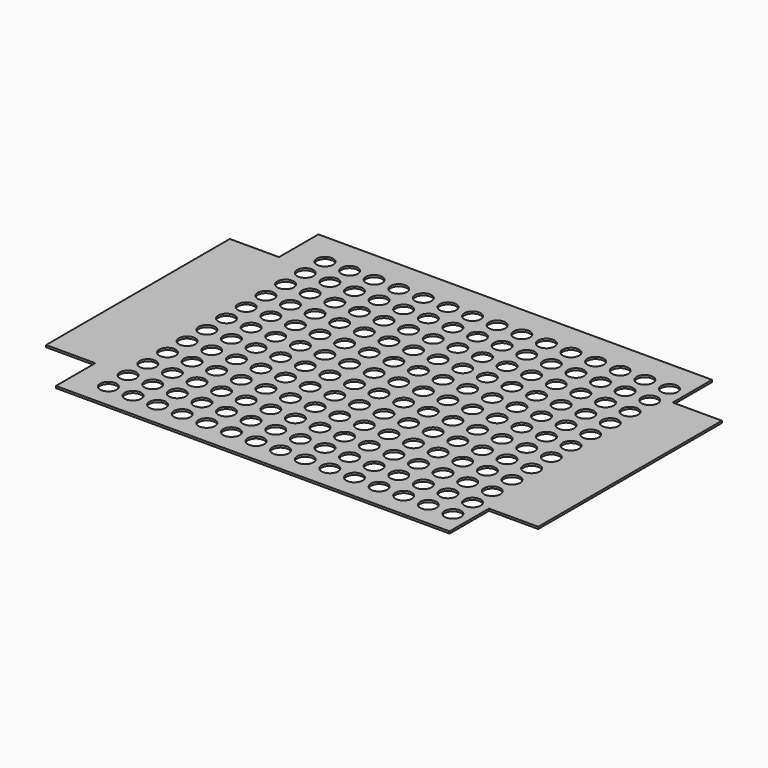
from build123d import *

# Parameters (mm, degrees)
F0_R     = 12.7
F1_DEPTH = 3.175


# Not quite as in the source:
# - a feature names something its author has since deleted; it is built from what else it names


with BuildPart() as f1:
    # F0 (on Top) → F1 (new body)
    with BuildSketch(Plane.XY):
        Polygon((-76.2, -76.2), (-76.2, 0), (-685.8, 0), (-685.8, -76.2), (-762, -76.2), (-762, -431.8), (-685.8, -431.8), (-685.8, -508), (-76.2, -508), (-76.2, -431.8), (0, -431.8), (0, -76.2), align=None)
        with Locations((-635, -469.9)):
            Circle(F0_R, mode=Mode.SUBTRACT)
        with Locations((-596.9, -469.9)):
            Circle(F0_R, mode=Mode.SUBTRACT)
        with Locations((-635, -431.8)):
            Circle(F0_R, mode=Mode.SUBTRACT)
        with Locations((-596.9, -431.8)):
            Circle(F0_R, mode=Mode.SUBTRACT)
        with Locations((-635, -393.7)):
            Circle(F0_R, mode=Mode.SUBTRACT)
        with Locations((-596.9, -393.7)):
            Circle(F0_R, mode=Mode.SUBTRACT)
        with Locations((-558.8, -469.9)):
            Circle(F0_R, mode=Mode.SUBTRACT)
        with Locations((-520.7, -469.9)):
            Circle(F0_R, mode=Mode.SUBTRACT)
        with Locations((-482.6, -469.9)):
            Circle(F0_R, mode=Mode.SUBTRACT)
        with Locations((-444.5, -469.9)):
            Circle(F0_R, mode=Mode.SUBTRACT)
        with Locations((-406.4, -469.9)):
            Circle(F0_R, mode=Mode.SUBTRACT)
        with Locations((-558.8, -431.8)):
            Circle(F0_R, mode=Mode.SUBTRACT)
        with Locations((-520.7, -431.8)):
            Circle(F0_R, mode=Mode.SUBTRACT)
        with Locations((-482.6, -431.8)):
            Circle(F0_R, mode=Mode.SUBTRACT)
        with Locations((-558.8, -393.7)):
            Circle(F0_R, mode=Mode.SUBTRACT)
        with Locations((-520.7, -393.7)):
            Circle(F0_R, mode=Mode.SUBTRACT)
        with Locations((-482.6, -393.7)):
            Circle(F0_R, mode=Mode.SUBTRACT)
        with Locations((-444.5, -431.8)):
            Circle(F0_R, mode=Mode.SUBTRACT)
        with Locations((-406.4, -431.8)):
            Circle(F0_R, mode=Mode.SUBTRACT)
        with Locations((-444.5, -393.7)):
            Circle(F0_R, mode=Mode.SUBTRACT)
        with Locations((-406.4, -393.7)):
            Circle(F0_R, mode=Mode.SUBTRACT)
        with Locations((-635, -355.6)):
            Circle(F0_R, mode=Mode.SUBTRACT)
        with Locations((-596.9, -355.6)):
            Circle(F0_R, mode=Mode.SUBTRACT)
        with Locations((-635, -317.5)):
            Circle(F0_R, mode=Mode.SUBTRACT)
        with Locations((-596.9, -317.5)):
            Circle(F0_R, mode=Mode.SUBTRACT)
        with Locations((-635, -279.4)):
            Circle(F0_R, mode=Mode.SUBTRACT)
        with Locations((-596.9, -279.4)):
            Circle(F0_R, mode=Mode.SUBTRACT)
        with Locations((-558.8, -355.6)):
            Circle(F0_R, mode=Mode.SUBTRACT)
        with Locations((-520.7, -355.6)):
            Circle(F0_R, mode=Mode.SUBTRACT)
        with Locations((-482.6, -355.6)):
            Circle(F0_R, mode=Mode.SUBTRACT)
        with Locations((-444.5, -355.6)):
            Circle(F0_R, mode=Mode.SUBTRACT)
        with Locations((-406.4, -355.6)):
            Circle(F0_R, mode=Mode.SUBTRACT)
        with Locations((-558.8, -317.5)):
            Circle(F0_R, mode=Mode.SUBTRACT)
        with Locations((-520.7, -317.5)):
            Circle(F0_R, mode=Mode.SUBTRACT)
        with Locations((-482.6, -317.5)):
            Circle(F0_R, mode=Mode.SUBTRACT)
        with Locations((-558.8, -279.4)):
            Circle(F0_R, mode=Mode.SUBTRACT)
        with Locations((-520.7, -279.4)):
            Circle(F0_R, mode=Mode.SUBTRACT)
        with Locations((-482.6, -279.4)):
            Circle(F0_R, mode=Mode.SUBTRACT)
        with Locations((-444.5, -317.5)):
            Circle(F0_R, mode=Mode.SUBTRACT)
        with Locations((-406.4, -317.5)):
            Circle(F0_R, mode=Mode.SUBTRACT)
        with Locations((-444.5, -279.4)):
            Circle(F0_R, mode=Mode.SUBTRACT)
        with Locations((-406.4, -279.4)):
            Circle(F0_R, mode=Mode.SUBTRACT)
        with Locations((-368.3, -469.9)):
            Circle(F0_R, mode=Mode.SUBTRACT)
        with Locations((-330.2, -469.9)):
            Circle(F0_R, mode=Mode.SUBTRACT)
        with Locations((-292.1, -469.9)):
            Circle(F0_R, mode=Mode.SUBTRACT)
        with Locations((-254, -469.9)):
            Circle(F0_R, mode=Mode.SUBTRACT)
        with Locations((-215.9, -469.9)):
            Circle(F0_R, mode=Mode.SUBTRACT)
        with Locations((-368.3, -431.8)):
            Circle(F0_R, mode=Mode.SUBTRACT)
        with Locations((-330.2, -431.8)):
            Circle(F0_R, mode=Mode.SUBTRACT)
        with Locations((-292.1, -431.8)):
            Circle(F0_R, mode=Mode.SUBTRACT)
        with Locations((-368.3, -393.7)):
            Circle(F0_R, mode=Mode.SUBTRACT)
        with Locations((-330.2, -393.7)):
            Circle(F0_R, mode=Mode.SUBTRACT)
        with Locations((-292.1, -393.7)):
            Circle(F0_R, mode=Mode.SUBTRACT)
        with Locations((-254, -431.8)):
            Circle(F0_R, mode=Mode.SUBTRACT)
        with Locations((-215.9, -431.8)):
            Circle(F0_R, mode=Mode.SUBTRACT)
        with Locations((-254, -393.7)):
            Circle(F0_R, mode=Mode.SUBTRACT)
        with Locations((-215.9, -393.7)):
            Circle(F0_R, mode=Mode.SUBTRACT)
        with Locations((-177.8, -469.9)):
            Circle(F0_R, mode=Mode.SUBTRACT)
        with Locations((-139.7, -469.9)):
            Circle(F0_R, mode=Mode.SUBTRACT)
        with Locations((-101.6, -469.9)):
            Circle(F0_R, mode=Mode.SUBTRACT)
        with Locations((-177.8, -431.8)):
            Circle(F0_R, mode=Mode.SUBTRACT)
        with Locations((-139.7, -431.8)):
            Circle(F0_R, mode=Mode.SUBTRACT)
        with Locations((-101.6, -431.8)):
            Circle(F0_R, mode=Mode.SUBTRACT)
        with Locations((-177.8, -393.7)):
            Circle(F0_R, mode=Mode.SUBTRACT)
        with Locations((-139.7, -393.7)):
            Circle(F0_R, mode=Mode.SUBTRACT)
        with Locations((-101.6, -393.7)):
            Circle(F0_R, mode=Mode.SUBTRACT)
        with Locations((-368.3, -355.6)):
            Circle(F0_R, mode=Mode.SUBTRACT)
        with Locations((-330.2, -355.6)):
            Circle(F0_R, mode=Mode.SUBTRACT)
        with Locations((-292.1, -355.6)):
            Circle(F0_R, mode=Mode.SUBTRACT)
        with Locations((-254, -355.6)):
            Circle(F0_R, mode=Mode.SUBTRACT)
        with Locations((-215.9, -355.6)):
            Circle(F0_R, mode=Mode.SUBTRACT)
        with Locations((-368.3, -317.5)):
            Circle(F0_R, mode=Mode.SUBTRACT)
        with Locations((-330.2, -317.5)):
            Circle(F0_R, mode=Mode.SUBTRACT)
        with Locations((-292.1, -317.5)):
            Circle(F0_R, mode=Mode.SUBTRACT)
        with Locations((-368.3, -279.4)):
            Circle(F0_R, mode=Mode.SUBTRACT)
        with Locations((-330.2, -279.4)):
            Circle(F0_R, mode=Mode.SUBTRACT)
        with Locations((-292.1, -279.4)):
            Circle(F0_R, mode=Mode.SUBTRACT)
        with Locations((-254, -317.5)):
            Circle(F0_R, mode=Mode.SUBTRACT)
        with Locations((-215.9, -317.5)):
            Circle(F0_R, mode=Mode.SUBTRACT)
        with Locations((-254, -279.4)):
            Circle(F0_R, mode=Mode.SUBTRACT)
        with Locations((-215.9, -279.4)):
            Circle(F0_R, mode=Mode.SUBTRACT)
        with Locations((-177.8, -355.6)):
            Circle(F0_R, mode=Mode.SUBTRACT)
        with Locations((-139.7, -355.6)):
            Circle(F0_R, mode=Mode.SUBTRACT)
        with Locations((-101.6, -355.6)):
            Circle(F0_R, mode=Mode.SUBTRACT)
        with Locations((-177.8, -317.5)):
            Circle(F0_R, mode=Mode.SUBTRACT)
        with Locations((-139.7, -317.5)):
            Circle(F0_R, mode=Mode.SUBTRACT)
        with Locations((-101.6, -317.5)):
            Circle(F0_R, mode=Mode.SUBTRACT)
        with Locations((-177.8, -279.4)):
            Circle(F0_R, mode=Mode.SUBTRACT)
        with Locations((-139.7, -279.4)):
            Circle(F0_R, mode=Mode.SUBTRACT)
        with Locations((-101.6, -279.4)):
            Circle(F0_R, mode=Mode.SUBTRACT)
        with Locations((-635, -241.3)):
            Circle(F0_R, mode=Mode.SUBTRACT)
        with Locations((-596.9, -241.3)):
            Circle(F0_R, mode=Mode.SUBTRACT)
        with Locations((-635, -203.2)):
            Circle(F0_R, mode=Mode.SUBTRACT)
        with Locations((-596.9, -203.2)):
            Circle(F0_R, mode=Mode.SUBTRACT)
        with Locations((-635, -165.1)):
            Circle(F0_R, mode=Mode.SUBTRACT)
        with Locations((-596.9, -165.1)):
            Circle(F0_R, mode=Mode.SUBTRACT)
        with Locations((-558.8, -241.3)):
            Circle(F0_R, mode=Mode.SUBTRACT)
        with Locations((-520.7, -241.3)):
            Circle(F0_R, mode=Mode.SUBTRACT)
        with Locations((-482.6, -241.3)):
            Circle(F0_R, mode=Mode.SUBTRACT)
        with Locations((-558.8, -203.2)):
            Circle(F0_R, mode=Mode.SUBTRACT)
        with Locations((-520.7, -203.2)):
            Circle(F0_R, mode=Mode.SUBTRACT)
        with Locations((-482.6, -203.2)):
            Circle(F0_R, mode=Mode.SUBTRACT)
        with Locations((-444.5, -241.3)):
            Circle(F0_R, mode=Mode.SUBTRACT)
        with Locations((-406.4, -241.3)):
            Circle(F0_R, mode=Mode.SUBTRACT)
        with Locations((-444.5, -203.2)):
            Circle(F0_R, mode=Mode.SUBTRACT)
        with Locations((-406.4, -203.2)):
            Circle(F0_R, mode=Mode.SUBTRACT)
        with Locations((-558.8, -165.1)):
            Circle(F0_R, mode=Mode.SUBTRACT)
        with Locations((-520.7, -165.1)):
            Circle(F0_R, mode=Mode.SUBTRACT)
        with Locations((-482.6, -165.1)):
            Circle(F0_R, mode=Mode.SUBTRACT)
        with Locations((-444.5, -165.1)):
            Circle(F0_R, mode=Mode.SUBTRACT)
        with Locations((-406.4, -165.1)):
            Circle(F0_R, mode=Mode.SUBTRACT)
        with Locations((-635, -127)):
            Circle(F0_R, mode=Mode.SUBTRACT)
        with Locations((-596.9, -127)):
            Circle(F0_R, mode=Mode.SUBTRACT)
        with Locations((-635, -88.9)):
            Circle(F0_R, mode=Mode.SUBTRACT)
        with Locations((-596.9, -88.9)):
            Circle(F0_R, mode=Mode.SUBTRACT)
        with Locations((-635, -50.8)):
            Circle(F0_R, mode=Mode.SUBTRACT)
        with Locations((-596.9, -50.8)):
            Circle(F0_R, mode=Mode.SUBTRACT)
        with Locations((-558.8, -127)):
            Circle(F0_R, mode=Mode.SUBTRACT)
        with Locations((-520.7, -127)):
            Circle(F0_R, mode=Mode.SUBTRACT)
        with Locations((-482.6, -127)):
            Circle(F0_R, mode=Mode.SUBTRACT)
        with Locations((-558.8, -88.9)):
            Circle(F0_R, mode=Mode.SUBTRACT)
        with Locations((-520.7, -88.9)):
            Circle(F0_R, mode=Mode.SUBTRACT)
        with Locations((-482.6, -88.9)):
            Circle(F0_R, mode=Mode.SUBTRACT)
        with Locations((-444.5, -127)):
            Circle(F0_R, mode=Mode.SUBTRACT)
        with Locations((-406.4, -127)):
            Circle(F0_R, mode=Mode.SUBTRACT)
        with Locations((-444.5, -88.9)):
            Circle(F0_R, mode=Mode.SUBTRACT)
        with Locations((-406.4, -88.9)):
            Circle(F0_R, mode=Mode.SUBTRACT)
        with Locations((-558.8, -50.8)):
            Circle(F0_R, mode=Mode.SUBTRACT)
        with Locations((-520.7, -50.8)):
            Circle(F0_R, mode=Mode.SUBTRACT)
        with Locations((-482.6, -50.8)):
            Circle(F0_R, mode=Mode.SUBTRACT)
        with Locations((-444.5, -50.8)):
            Circle(F0_R, mode=Mode.SUBTRACT)
        with Locations((-406.4, -50.8)):
            Circle(F0_R, mode=Mode.SUBTRACT)
        with Locations((-368.3, -241.3)):
            Circle(F0_R, mode=Mode.SUBTRACT)
        with Locations((-330.2, -241.3)):
            Circle(F0_R, mode=Mode.SUBTRACT)
        with Locations((-292.1, -241.3)):
            Circle(F0_R, mode=Mode.SUBTRACT)
        with Locations((-368.3, -203.2)):
            Circle(F0_R, mode=Mode.SUBTRACT)
        with Locations((-330.2, -203.2)):
            Circle(F0_R, mode=Mode.SUBTRACT)
        with Locations((-292.1, -203.2)):
            Circle(F0_R, mode=Mode.SUBTRACT)
        with Locations((-254, -241.3)):
            Circle(F0_R, mode=Mode.SUBTRACT)
        with Locations((-215.9, -241.3)):
            Circle(F0_R, mode=Mode.SUBTRACT)
        with Locations((-254, -203.2)):
            Circle(F0_R, mode=Mode.SUBTRACT)
        with Locations((-215.9, -203.2)):
            Circle(F0_R, mode=Mode.SUBTRACT)
        with Locations((-368.3, -165.1)):
            Circle(F0_R, mode=Mode.SUBTRACT)
        with Locations((-330.2, -165.1)):
            Circle(F0_R, mode=Mode.SUBTRACT)
        with Locations((-292.1, -165.1)):
            Circle(F0_R, mode=Mode.SUBTRACT)
        with Locations((-254, -165.1)):
            Circle(F0_R, mode=Mode.SUBTRACT)
        with Locations((-215.9, -165.1)):
            Circle(F0_R, mode=Mode.SUBTRACT)
        with Locations((-177.8, -241.3)):
            Circle(F0_R, mode=Mode.SUBTRACT)
        with Locations((-139.7, -241.3)):
            Circle(F0_R, mode=Mode.SUBTRACT)
        with Locations((-101.6, -241.3)):
            Circle(F0_R, mode=Mode.SUBTRACT)
        with Locations((-177.8, -203.2)):
            Circle(F0_R, mode=Mode.SUBTRACT)
        with Locations((-139.7, -203.2)):
            Circle(F0_R, mode=Mode.SUBTRACT)
        with Locations((-101.6, -203.2)):
            Circle(F0_R, mode=Mode.SUBTRACT)
        with Locations((-177.8, -165.1)):
            Circle(F0_R, mode=Mode.SUBTRACT)
        with Locations((-139.7, -165.1)):
            Circle(F0_R, mode=Mode.SUBTRACT)
        with Locations((-101.6, -165.1)):
            Circle(F0_R, mode=Mode.SUBTRACT)
        with Locations((-368.3, -127)):
            Circle(F0_R, mode=Mode.SUBTRACT)
        with Locations((-330.2, -127)):
            Circle(F0_R, mode=Mode.SUBTRACT)
        with Locations((-292.1, -127)):
            Circle(F0_R, mode=Mode.SUBTRACT)
        with Locations((-368.3, -88.9)):
            Circle(F0_R, mode=Mode.SUBTRACT)
        with Locations((-330.2, -88.9)):
            Circle(F0_R, mode=Mode.SUBTRACT)
        with Locations((-292.1, -88.9)):
            Circle(F0_R, mode=Mode.SUBTRACT)
        with Locations((-254, -127)):
            Circle(F0_R, mode=Mode.SUBTRACT)
        with Locations((-215.9, -127)):
            Circle(F0_R, mode=Mode.SUBTRACT)
        with Locations((-254, -88.9)):
            Circle(F0_R, mode=Mode.SUBTRACT)
        with Locations((-215.9, -88.9)):
            Circle(F0_R, mode=Mode.SUBTRACT)
        with Locations((-368.3, -50.8)):
            Circle(F0_R, mode=Mode.SUBTRACT)
        with Locations((-330.2, -50.8)):
            Circle(F0_R, mode=Mode.SUBTRACT)
        with Locations((-292.1, -50.8)):
            Circle(F0_R, mode=Mode.SUBTRACT)
        with Locations((-254, -50.8)):
            Circle(F0_R, mode=Mode.SUBTRACT)
        with Locations((-215.9, -50.8)):
            Circle(F0_R, mode=Mode.SUBTRACT)
        with Locations((-177.8, -127)):
            Circle(F0_R, mode=Mode.SUBTRACT)
        with Locations((-139.7, -127)):
            Circle(F0_R, mode=Mode.SUBTRACT)
        with Locations((-101.6, -127)):
            Circle(F0_R, mode=Mode.SUBTRACT)
        with Locations((-177.8, -88.9)):
            Circle(F0_R, mode=Mode.SUBTRACT)
        with Locations((-139.7, -88.9)):
            Circle(F0_R, mode=Mode.SUBTRACT)
        with Locations((-101.6, -88.9)):
            Circle(F0_R, mode=Mode.SUBTRACT)
        with Locations((-177.8, -50.8)):
            Circle(F0_R, mode=Mode.SUBTRACT)
        with Locations((-139.7, -50.8)):
            Circle(F0_R, mode=Mode.SUBTRACT)
        with Locations((-101.6, -50.8)):
            Circle(F0_R, mode=Mode.SUBTRACT)
    extrude(amount=F1_DEPTH)


solid = f1.part
